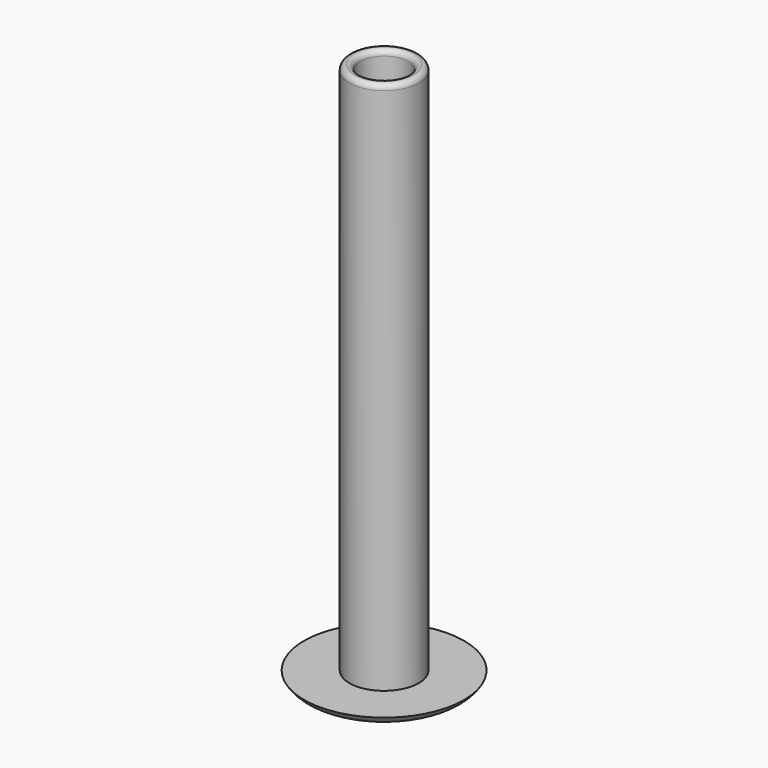
from build123d import *

# Parameters (mm, degrees)
F0_R     = 3.25
F0_R_2   = 2.25
F1_DEPTH = 51
F0_R_3   = 7.5
F2_DEPTH = 1
F3_R     = 0.49999
F5_R     = 1


# Not quite as in the source:
# - a fillet or chamfer that OpenCascade refuses, or shapes differently, is made with other operations: its cross-section is extruded or revolved along the edge and cut away or added
# - a fillet or chamfer is up to 0.001 mm smaller than in the source, because OpenCascade refuses the exact size


with BuildPart() as f1:
    # F0 (on Top) → F1 (new body)
    with BuildSketch(Plane.XY):
        Circle(F0_R)
        Circle(F0_R_2, mode=Mode.SUBTRACT)
    extrude(amount=F1_DEPTH)

    # F0 (on Top) → F2 (join)
    with BuildSketch(Plane.XY):
        Circle(F0_R_3)
        Circle(F0_R, mode=Mode.SUBTRACT)
    extrude(amount=F2_DEPTH)

    # F3 (radius 0.5 in the source; OpenCascade refuses exactly that, so slightly less here)
    f3_edges = [f1.edges().sort_by_distance(p)[0] for p in [
        (-3.25, 0, 51),
        (-2.25, 0, 51),
    ]]
    fillet(f3_edges, radius=F3_R)

    # F4: fillet of radius 2 on 1 edges, made by hand

    # F4_s1 → F4_t2 (revolve, cut)
    with BuildSketch(Plane.XZ):
        with BuildLine():
            ThreePointArc((7.5, 1), (6.7679491924, 0.2679491924), (5.7679491924, 0))
            Line((5.7679491924, 0), (7.5, 0))
            Line((7.5, 0), (7.5, 1))
        make_face()
    revolve(axis=Axis((0, 0, 0), (0, 0, 1)), mode=Mode.SUBTRACT)

    # F5
    f5_edges = [f1.edges().sort_by_distance(p)[0] for p in [
        (-2.25, 0, 0),
    ]]
    fillet(f5_edges, radius=F5_R)


solid = f1.part
